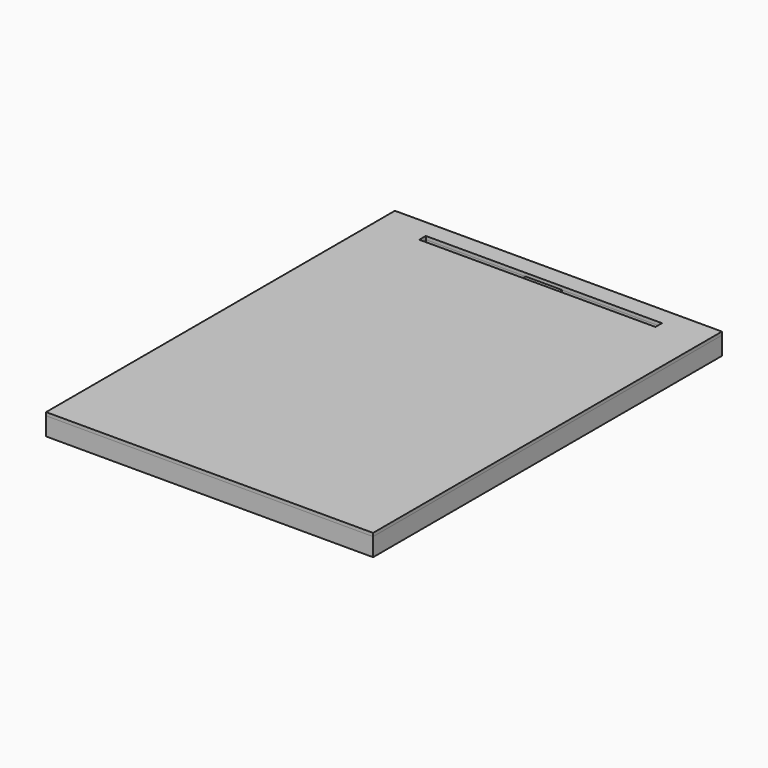
from build123d import *

# Parameters (mm, degrees)
F0_W     = 525
F0_H     = 50
F0_W_2   = 200
F0_H_2   = 45
F1_DEPTH = 100
F0_H_3   = 1125
F0_H_4   = 980
F2_DEPTH = 18


# Not quite as in the source:
# - a feature names something its author has since deleted; it is built from what else it names


with BuildPart() as f1:
    # F0 (on Top) → F1 (new body)
    with BuildSketch(Plane.XY):
        Polygon((850, -1150), (900, -1150), (900, 1150), (850, 1150), (850, 1100), (850, 1055), (850, 1005), (850, 25), (850, -25), align=None)
        Polygon((-900, -1200), (900, -1200), (900, -1150), (850, -1150), (325, -1150), (275, -1150), (-275, -1150), (-325, -1150), (-850, -1150), (-900, -1150), align=None)
        Polygon((-900, 1150), (-900, -1150), (-850, -1150), (-850, -25), (-850, 25), (-850, 1005), (-850, 1055), (-850, 1100), (-850, 1150), align=None)
        with Locations((-587.5, 0)):
            Rectangle(F0_W, F0_H)
        Polygon((0, -25), (275, -25), (275, 25), (0, 25), (-275, 25), (-275, -25), align=None)
        Polygon((275, -1150), (325, -1150), (325, -25), (325, 25), (325, 1005), (275, 1005), (275, 25), (275, -25), align=None)
        with Locations((587.5, 0)):
            Rectangle(F0_W, F0_H)
        Polygon((850, 1150), (900, 1150), (900, 1200), (-900, 1200), (-900, 1150), (-850, 1150), align=None)
        Polygon((850, 1005), (850, 1055), (650, 1055), (100, 1055), (-100, 1055), (-650, 1055), (-850, 1055), (-850, 1005), (-325, 1005), (-275, 1005), (275, 1005), (325, 1005), align=None)
        Polygon((850, 1100), (850, 1150), (-850, 1150), (-850, 1100), (-650, 1100), (-100, 1100), (100, 1100), (650, 1100), align=None)
        with Locations((-750, 1077.5)):
            Rectangle(F0_W_2, F0_H_2)
        with Locations((0, 1077.5)):
            Rectangle(F0_W_2, F0_H_2)
        with Locations((750, 1077.5)):
            Rectangle(F0_W_2, F0_H_2)
        Polygon((-325, -25), (-325, -1150), (-275, -1150), (-275, -25), (-275, 25), (-275, 1005), (-325, 1005), (-325, 25), align=None)
    extrude(amount=-F1_DEPTH)


with BuildPart() as f2:
    # F0 (on Top) → F2 (new body)
    with BuildSketch(Plane.XY):
        with Locations((-587.5, -587.5)):
            Rectangle(F0_W, F0_H_3)
        Polygon((-275, -1150), (275, -1150), (275, -25), (0, -25), (-275, -25), align=None)
        with Locations((587.5, -587.5)):
            Rectangle(F0_W, F0_H_3)
        with Locations((-587.5, 515)):
            Rectangle(F0_W, F0_H_4)
        Polygon((0, 25), (275, 25), (275, 1005), (-275, 1005), (-275, 25), align=None)
        with Locations((587.5, 515)):
            Rectangle(F0_W, F0_H_4)
        with Locations((750, 1077.5)):
            Rectangle(F0_W_2, F0_H_2)
        Polygon((850, -1150), (900, -1150), (900, 1150), (850, 1150), (850, 1100), (850, 1055), (850, 1005), (850, 25), (850, -25), align=None)
        Polygon((850, 1150), (900, 1150), (900, 1200), (-900, 1200), (-900, 1150), (-850, 1150), align=None)
        Polygon((850, 1100), (850, 1150), (-850, 1150), (-850, 1100), (-650, 1100), (-100, 1100), (100, 1100), (650, 1100), align=None)
        Polygon((-900, 1150), (-900, -1150), (-850, -1150), (-850, -25), (-850, 25), (-850, 1005), (-850, 1055), (-850, 1100), (-850, 1150), align=None)
        with Locations((-750, 1077.5)):
            Rectangle(F0_W_2, F0_H_2)
        Polygon((850, 1005), (850, 1055), (650, 1055), (100, 1055), (-100, 1055), (-650, 1055), (-850, 1055), (-850, 1005), (-325, 1005), (-275, 1005), (275, 1005), (325, 1005), align=None)
        with Locations((-587.5, 0)):
            Rectangle(F0_W, F0_H)
        Polygon((0, -25), (275, -25), (275, 25), (0, 25), (-275, 25), (-275, -25), align=None)
        Polygon((275, -1150), (325, -1150), (325, -25), (325, 25), (325, 1005), (275, 1005), (275, 25), (275, -25), align=None)
        with Locations((587.5, 0)):
            Rectangle(F0_W, F0_H)
        Polygon((-900, -1200), (900, -1200), (900, -1150), (850, -1150), (325, -1150), (275, -1150), (-275, -1150), (-325, -1150), (-850, -1150), (-900, -1150), align=None)
        Polygon((-325, -25), (-325, -1150), (-275, -1150), (-275, -25), (-275, 25), (-275, 1005), (-325, 1005), (-325, 25), align=None)
    extrude(amount=F2_DEPTH)


solid = Compound([f1.part, f2.part])
